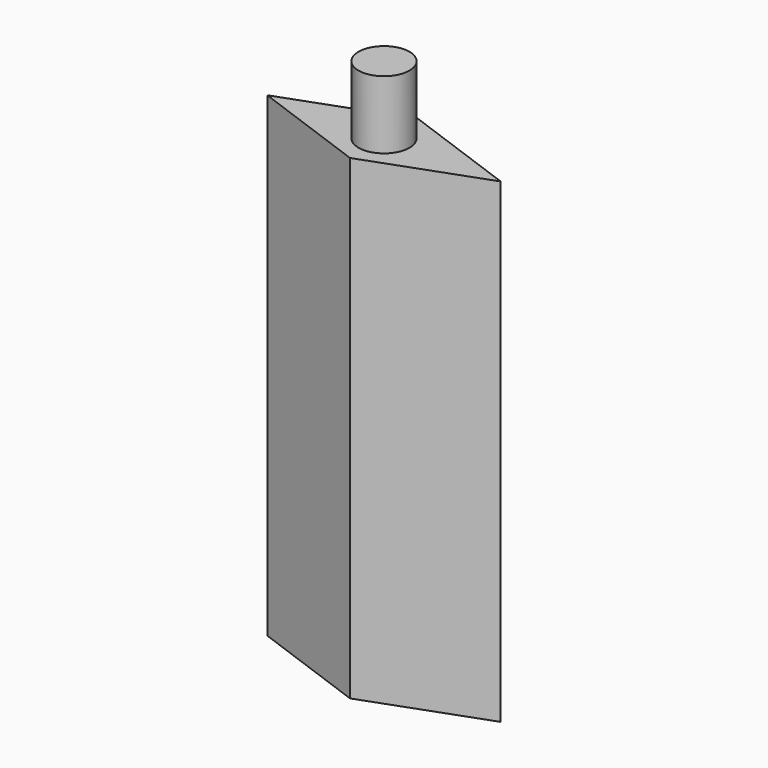
from build123d import *

# Parameters (mm, degrees)
F0_W        = 101.6
F0_H        = 31.75
F1_DEPTH    = 177.8
F2_T1_DEPTH = 441.3701848271
F3_R        = 9.525
F4_DEPTH    = 25.4
F5_R        = 9.525
F6_DEPTH    = 25.4


# Not quite as in the source:
# - a fillet or chamfer that OpenCascade refuses, or shapes differently, is made with other operations: its cross-section is extruded or revolved along the edge and cut away or added


with BuildPart() as f1:
    # F0 (on Top) → F1 (new body)
    with BuildSketch(Plane.XY):
        Rectangle(F0_W, F0_H)
    extrude(amount=F1_DEPTH)

    # F2: chamfer of 50.8 x 18.4896879007 on 4 edges, made by hand

    # F2_s2 → F2_t1 (cut)
    with BuildSketch(Plane.XY.offset(-131.7850924136)):
        Polygon((50.8, -2.6146879007), (0, 15.875), (50.8, 15.875), align=None)
        Polygon((50.8, 2.6146879007), (0, -15.875), (50.8, -15.875), align=None)
        Polygon((-50.8, 2.6146879007), (0, -15.875), (-50.8, -15.875), align=None)
        Polygon((0, 15.875), (-50.8, -2.6146879007), (-50.8, 15.875), align=None)
    extrude(amount=F2_T1_DEPTH, mode=Mode.SUBTRACT)

    # F3 (on face) → F4 (join)
    with BuildSketch(Plane.XY.offset(177.8)):
        Circle(F3_R)
    extrude(amount=F4_DEPTH)

    # F5 (on face) → F6 (cut)
    with BuildSketch(Plane(origin=(0, 0, 0), x_dir=(1, 0, 0), z_dir=(0, 0, -1))):
        Circle(F5_R)
    extrude(amount=-F6_DEPTH, mode=Mode.SUBTRACT)


solid = f1.part
